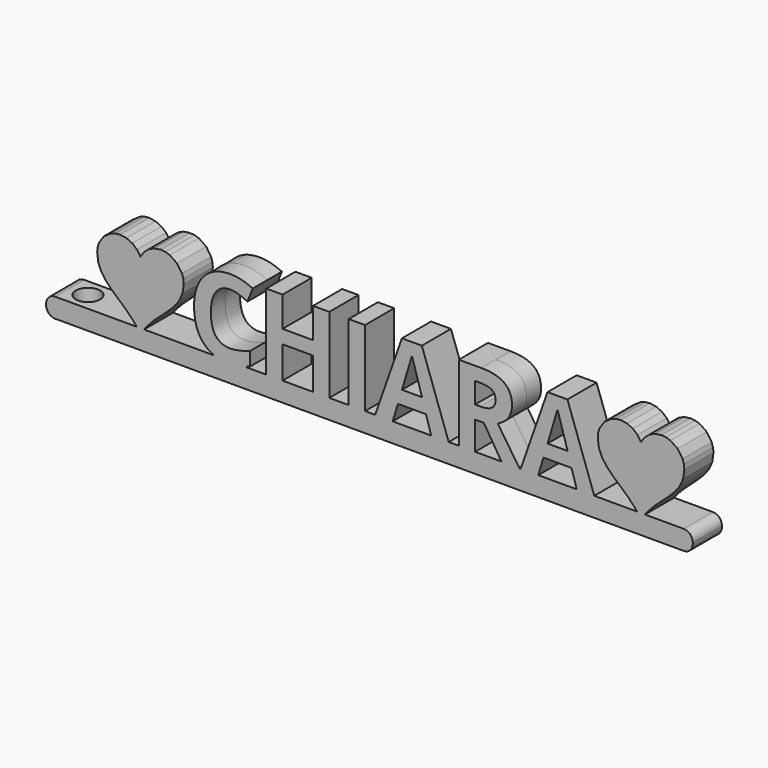
from build123d import *

# Parameters (mm, degrees)
F0_TEXT_SIZE = 17.7567247505
F1_DEPTH     = 3
F2_W         = 99
F2_H         = 6
F3_DEPTH     = 0.2
F4_DEPTH     = 3
F5_W         = 6
F5_H         = 3.2
F6_DEPTH     = 7.5
F7_R         = 1.5
F8_R         = 2
F9_DEPTH     = 4
F10_R        = 1.5


# Not quite as in the source:
# - Text() gives the source's letters only with a copy of the font that has no kerning and outlines rounded to 1/6400 em; it was checked with that copy


with BuildPart() as f1:
    # F0 (on Front) → F1 (new body, symmetric)
    with BuildSketch(Plane.XZ):
        Polygon((67.1837163837, 12.4433699982), (66.1226963837, 12.5970599982), (65.3640863837, 12.5204799982), (64.6572863837, 12.3008699982), (63.4599463837, 11.4933499982), (62.6523263837, 10.2961199982), (62.4326763837, 9.5893599982), (62.3560863837, 8.8307599982), (62.5446063837, 7.3860999982), (63.0653463837, 6.1597099982), (63.8510963837, 5.0814099982), (64.8346263837, 4.0810299982), (67.1314763837, 2.0250499982), (68.3160663837, 0.8247399982), (69.4390563837, -0.5860800018), (69.4833363837, -0.6500000018), (69.5263663837, -0.5851400018), (70.6042763837, 0.8234499982), (71.7675763837, 2.0333299982), (74.0712463837, 4.1212499982), (75.0720363837, 5.1327499982), (75.8770363837, 6.2116199982), (76.4134263837, 7.4226699982), (76.6084063837, 8.8307599982), (76.5318263837, 9.5893599982), (76.3122163837, 10.2961199982), (75.5046963837, 11.4933499982), (74.3074663837, 12.3008699982), (73.6006963837, 12.5204799982), (72.8421063837, 12.5970599982), (71.7810863837, 12.4433699982), (70.8400163837, 12.0123599982), (70.0600663837, 11.3491699982), (69.4823963837, 10.4989199982), (68.9047363837, 11.3491699982), (68.1247863837, 12.0123599982), align=None)
        Polygon((-15.2581707838, 12.5082299799), (-16.3191907838, 12.6619199799), (-17.0778007838, 12.5853399799), (-17.7846007838, 12.3657299799), (-18.9819407838, 11.5582099799), (-19.7895607838, 10.3609799799), (-20.0092107838, 9.6542199799), (-20.0858007838, 8.8956199799), (-19.8972807838, 7.4509599799), (-19.3765407838, 6.2245699799), (-18.5907907838, 5.1462699799), (-17.6072607838, 4.1458899799), (-15.3104107838, 2.0899099799), (-14.1258207838, 0.8895999799), (-13.0028307838, -0.5212200201), (-12.9585507838, -0.5851400201), (-12.9155207838, -0.5202800201), (-11.8376107838, 0.8883099799), (-10.6743107838, 2.0981899799), (-8.3706407838, 4.1861099799), (-7.3698507838, 5.1976099799), (-6.5648507838, 6.2764799799), (-6.0284607838, 7.4875299799), (-5.8334807838, 8.8956199799), (-5.9100607838, 9.6542199799), (-6.1296707838, 10.3609799799), (-6.9371907838, 11.5582099799), (-8.1344207838, 12.3657299799), (-8.8411907838, 12.5853399799), (-9.5997807838, 12.6619199799), (-10.6608007838, 12.5082299799), (-11.6018707838, 12.0772199799), (-12.3818207838, 11.4140299799), (-12.9594907838, 10.5637799799), (-13.5371507838, 11.4140299799), (-14.3171007838, 12.0772199799), align=None)
        with Locations((-5.1580781594, 0)):
            Text('CHIARA', F0_TEXT_SIZE, font='Open Sans', font_style=FontStyle.BOLD, text_align=(TextAlign.LEFT, TextAlign.BOTTOM))
    extrude(amount=F1_DEPTH, both=True)



with BuildPart() as f3:
    # F2 (on Top) → F3 (new body)
    with BuildSketch(Plane.XY):
        with Locations((28.5, 0)):
            Rectangle(F2_W, F2_H)
    extrude(amount=F3_DEPTH)


with BuildPart() as f4:
    # F4 (new): a face of the model
    f4_faces = [f3.part.faces().sort_by_distance(p)[0] for p in [
        (28.5, 0, 0),
    ]]
    extrude(f4_faces, amount=F4_DEPTH)


with BuildPart() as f1_1:
    add(f1.part)

    add(f3.part)  # F6 merges F3

    add(f4.part)  # F6 merges F4
    # F5 (on face) → F6 (join)
    with BuildSketch(Plane(origin=(-21, 0, 0), x_dir=(0, -1, 0), z_dir=(-1, 0, 0))):
        with Locations((0, -1.4)):
            Rectangle(F5_W, F5_H)
    extrude(amount=F6_DEPTH)

    # F7
    f7_edges = [f1_1.edges().sort_by_distance(p)[0] for p in [
        (-28.5, 0, -3),
        (-28.5, 0, 0.2),
        (78, 0, -3),
    ]]
    fillet(f7_edges, radius=F7_R)

    # F8 (on face) → F9 (cut)
    with BuildSketch(Plane.XY.offset(0.2)):
        with Locations((-24, 0)):
            Circle(F8_R)
    extrude(amount=-F9_DEPTH, mode=Mode.SUBTRACT)

    # F10
    f10_edges = [f1_1.edges().sort_by_distance(p)[0] for p in [
        (78, 0, 0.2),
    ]]
    fillet(f10_edges, radius=F10_R)


solid = f1_1.part
